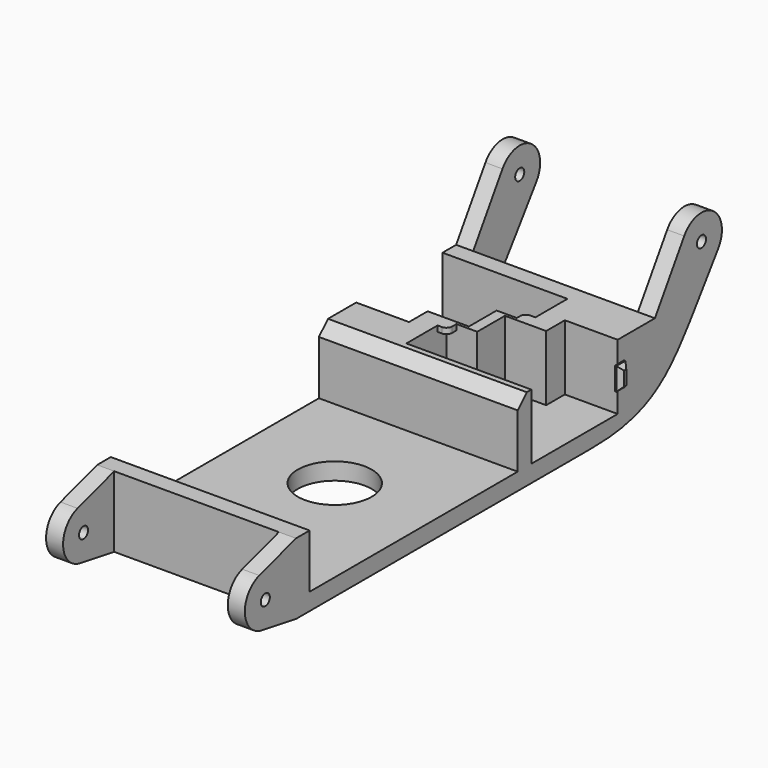
from build123d import *

# Parameters (mm, degrees)
F0_R      = 6.5
F0_W      = 34.999999702
F0_H      = 3
F0_H_2    = 0.3
F1_DEPTH  = 3
F2_DEPTH  = 9.5
F3_DEPTH  = 11.5
F5_DEPTH  = 3
F7_DEPTH  = 3
F8_R      = 1
F9_DEPTH  = 35.000999702
F11_DEPTH = 1
F13_DEPTH = 1
F14_SIZE  = 0.75
F15_W     = 1.8819853365
F15_H     = 1.731043148
F15_W_2   = 1.7636035271
F15_H_2   = 1.938064149
F16_DEPTH = 1
F18_DEPTH = 36.000999702
F19_R     = 1
F20_SIZE2 = 2
F20_SIZE  = 2


# Not quite as in the source:
# - ends of sketch curves that miss each other by under 0.0002 mm in the source are joined
# - a feature names something its author has since deleted; it is built from what else it names


with BuildPart() as f1:
    # F0 (on Top) → F1 (new body)
    with BuildSketch(Plane.XY):
        Polygon((7.8607099131, 16.1003852367), (-9.6392899379, 16.1003852367), (-9.6392899379, -29.3996147633), (25.3607097641, -29.3996147633), (25.3607097641, 16.1003852367), align=None)
        with Locations((7.8607099131, -2.2867515218)):
            Circle(F0_R, mode=Mode.SUBTRACT)
        with Locations((7.8607099131, -31.1996147633)):
            Rectangle(F0_W, F0_H)
        Polygon((-9.6392899379, 19.1003852367), (-9.6392899379, 16.1003852367), (7.8607099131, 16.1003852367), (25.3607097641, 16.1003852367), (25.3607097641, 19.1003852367), (22.192974557, 19.1003852367), (3.3607097641, 19.1003852367), align=None)
        Polygon((-9.6392899379, 46.3003852367), (-9.6392899379, 43.3003852367), (-6.4715547308, 43.3003852367), (12.3607100621, 43.3003852367), (25.3607097641, 43.3003852367), (25.3607097641, 46.3003852367), align=None)
        with Locations((7.8607099131, -29.5496147633)):
            Rectangle(F0_W, F0_H_2)
        Polygon((16.0607097641, 38.1003852367), (25.3607097641, 38.1003852367), (25.3607097641, 43.3003852367), (12.3607100621, 43.3003852367), (12.3607100621, 35.3003852367), (12.3607100621, 34.5003852367), (7.8607097641, 34.5003852367), (7.8607100621, 33.9926332235), (8.7954637781, 33.9926332235), (16.0607097641, 33.9926332235), align=None)
        Polygon((-9.6392899379, 24.3003852367), (-9.6392899379, 19.1003852367), (3.3607097641, 19.1003852367), (3.3607097641, 27.1003852367), (3.3607097641, 27.9003852367), (7.8607100621, 27.9003852367), (7.8607100621, 28.4081372499), (6.9259563461, 28.4081372499), (-0.3392899379, 28.4081372499), (-0.3392899379, 24.3003852367), align=None)
        Polygon((6.9259563461, 34.5003852367), (6.9259563461, 28.4081372499), (7.8607097641, 28.4081372499), (7.8607100621, 33.9926332235), (7.8607100621, 34.5003852367), align=None)
        Polygon((7.8607100621, 28.4081372499), (7.8607100621, 27.9003852367), (8.7954637781, 27.9003852367), (8.7954637781, 33.9926332235), (7.8607097641, 33.9926332235), align=None)
        Polygon((-9.6392899379, 43.3003852367), (-9.6392899379, 24.3003852367), (-0.3392899379, 24.3003852367), (-0.3392899379, 28.4081372499), (6.9259563461, 28.4081372499), (6.9259563461, 34.5003852367), (7.8607100621, 34.5003852367), (12.3607100621, 34.5003852367), (12.3607100621, 35.3003852367), (12.3607100621, 43.3003852367), (-6.4715547308, 43.3003852367), align=None)
        Polygon((3.3607097641, 27.1003852367), (3.3607097641, 19.1003852367), (22.192974557, 19.1003852367), (25.3607097641, 19.1003852367), (25.3607097641, 38.1003852367), (16.0607097641, 38.1003852367), (16.0607097641, 33.9926332235), (8.7954637781, 33.9926332235), (8.7954637781, 27.9003852367), (7.8607100621, 27.9003852367), (3.3607097641, 27.9003852367), align=None)
    extrude(amount=-F1_DEPTH)

    # F0 (on Top) → F2 (join)
    with BuildSketch(Plane.XY):
        with Locations((7.8607099131, -31.1996147633)):
            Rectangle(F0_W, F0_H)
        Polygon((-9.6392899379, 19.1003852367), (-9.6392899379, 16.1003852367), (7.8607099131, 16.1003852367), (25.3607097641, 16.1003852367), (25.3607097641, 19.1003852367), (22.192974557, 19.1003852367), (3.3607097641, 19.1003852367), align=None)
    extrude(amount=F2_DEPTH)

    # F0 (on Top) → F3 (join)
    with BuildSketch(Plane.XY):
        Polygon((-9.6392899379, 46.3003852367), (-9.6392899379, 43.3003852367), (-6.4715547308, 43.3003852367), (12.3607100621, 43.3003852367), (25.3607097641, 43.3003852367), (25.3607097641, 46.3003852367), align=None)
        Polygon((-9.6392899379, 24.3003852367), (-9.6392899379, 19.1003852367), (3.3607097641, 19.1003852367), (3.3607097641, 27.1003852367), (3.3607097641, 27.9003852367), (7.8607100621, 27.9003852367), (7.8607100621, 28.4081372499), (6.9259563461, 28.4081372499), (-0.3392899379, 28.4081372499), (-0.3392899379, 24.3003852367), align=None)
        Polygon((7.8607100621, 28.4081372499), (7.8607100621, 27.9003852367), (8.7954637781, 27.9003852367), (8.7954637781, 33.9926332235), (7.8607097641, 33.9926332235), align=None)
        Polygon((6.9259563461, 34.5003852367), (6.9259563461, 28.4081372499), (7.8607097641, 28.4081372499), (7.8607100621, 33.9926332235), (7.8607100621, 34.5003852367), align=None)
        Polygon((16.0607097641, 38.1003852367), (25.3607097641, 38.1003852367), (25.3607097641, 43.3003852367), (12.3607100621, 43.3003852367), (12.3607100621, 35.3003852367), (12.3607100621, 34.5003852367), (7.8607097641, 34.5003852367), (7.8607100621, 33.9926332235), (8.7954637781, 33.9926332235), (16.0607097641, 33.9926332235), align=None)
        Polygon((-9.6392899379, 19.1003852367), (-9.6392899379, 16.1003852367), (7.8607099131, 16.1003852367), (25.3607097641, 16.1003852367), (25.3607097641, 19.1003852367), (22.192974557, 19.1003852367), (3.3607097641, 19.1003852367), align=None)
    extrude(amount=F3_DEPTH)

    # F4 (on face) → F5 (join)
    with BuildSketch(Plane.YZ.offset(25.3607097641)):
        Polygon((-32.6996147633, -3), (46.3003852367, -3), (46.3003852367, 11.5), (38.1003852367, 11.5), (38.1003852367, 0), (19.1003852367, 0), (19.1003852367, 11.5), (16.1003852367, 11.5), (16.1003852367, 0), (-29.6996147633, 0), (-29.6996147633, 9.5), (-32.6996147633, 9.5), align=None)
        with BuildLine():
            Line((46.3003852367, 11.5), (46.3003852367, -3))
            Line((46.3003852367, -3), (60.2135883006, 16.6053474951))
            ThreePointArc((60.2135883006, 16.6053474951), (54.0324103863, 15.4756413664), (52.7478740756, 21.6265082006))
            Line((52.7478740756, 21.6265082006), (46.3003852367, 11.5))
        make_face()
        with BuildLine():
            ThreePointArc((52.7478740756, 21.6265082006), (54.0324103863, 15.4756413664), (60.2135883006, 16.6053474951))
            ThreePointArc((60.2135883006, 16.6053474951), (60.8312132136, 17.8429507129), (61.0437823534, 19.2096754909))
            ThreePointArc((61.0437823534, 19.2096754909), (57.8024349564, 23.5300682537), (52.7478740756, 21.6265082006))
        make_face()
        with BuildLine():
            Line((-40.2101505455, -1.7121333681), (-32.6996147633, -3))
            Line((-32.6996147633, -3), (-32.6996147633, 9.5))
            Line((-32.6996147633, 9.5), (-40.7689799002, 7.0253734949))
            ThreePointArc((-40.7689799002, 7.0253734949), (-36.7744645914, 6.3416367755), (-34.9496147633, 2.7231327258))
            ThreePointArc((-34.9496147633, 2.7231327258), (-36.5489606146, -0.7172459612), (-40.2101505455, -1.7121333681))
        make_face()
        with BuildLine():
            ThreePointArc((-40.7689799002, 7.0253734949), (-43.9404391312, 2.4359106929), (-40.2101505455, -1.7121333681))
            ThreePointArc((-40.2101505455, -1.7121333681), (-36.5489606146, -0.7172459612), (-34.9496147633, 2.7231327258))
            ThreePointArc((-34.9496147633, 2.7231327258), (-36.7744645914, 6.3416367755), (-40.7689799002, 7.0253734949))
        make_face()
    extrude(amount=-F5_DEPTH)

    # F6 (on face) → F7 (join)
    with BuildSketch(Plane(origin=(-9.6392899379, 0, 0), x_dir=(0, -1, 0), z_dir=(-1, 0, 0))):
        with BuildLine():
            Line((-60.2135883006, 16.6053474951), (-46.3003852367, -3))
            Line((-46.3003852367, -3), (-46.3003852367, 11.5))
            Line((-46.3003852367, 11.5), (-52.7478740756, 21.6265082006))
            ThreePointArc((-52.7478740756, 21.6265082006), (-59.0551543205, 22.9437096154), (-60.2135883006, 16.6053474951))
        make_face()
        Polygon((-46.3003852367, 11.5), (-46.3003852367, -3), (32.6996147633, -3), (32.6996147633, 9.5), (29.6996147633, 9.5), (29.6996147633, 0), (-16.1003852367, 0), (-16.1003852367, 11.5), (-24.3003852367, 11.5), (-24.3003852367, 0), (-43.3003852367, 0), (-43.3003852367, 11.5), align=None)
        with BuildLine():
            Line((32.6996147633, 9.5), (32.6996147633, -3))
            Line((32.6996147633, -3), (40.2101505455, -1.7121333681))
            ThreePointArc((40.2101505455, -1.7121333681), (43.9404391312, 2.4359106929), (40.7689799002, 7.0253734949))
            Line((40.7689799002, 7.0253734949), (32.6996147633, 9.5))
        make_face()
    extrude(amount=-F7_DEPTH)

    # F8 (on face) → F9 (cut, through all)
    with BuildSketch(Plane(origin=(-9.6392899379, 0, 0), x_dir=(0, -1, 0), z_dir=(-1, 0, 0))):
        with Locations((-56.5437823534, 19.2096754909)):
            Circle(F8_R)
        with Locations((39.4496147633, 2.7231327258)):
            Circle(F8_R)
    extrude(amount=-F9_DEPTH, mode=Mode.SUBTRACT)

    # F10 (on face) → F11 (join)
    with BuildSketch(Plane.YZ.offset(25.3607097641)):
        Polygon((39.4906885922, 7.75), (38.1003852367, 7.75), (38.1003852367, 3.75), (39.4906885922, 3.75), (39.4906885922, 5.75), align=None)
        Polygon((38.1003852367, 3.75), (38.1003852367, 7.75), (37.4906885922, 7.75), (37.4906885922, 5.75), (37.4906885922, 3.75), align=None)
    extrude(amount=F11_DEPTH)

    # F12 (on face) → F13 (join)
    with BuildSketch(Plane(origin=(-9.6392899379, 0, 0), x_dir=(0, -1, 0), z_dir=(-1, 0, 0))):
        Polygon((-22.9083076119, 7.75), (-24.3003852367, 7.75), (-24.3003852367, 3.75), (-22.9083076119, 3.75), (-22.9083076119, 5.75), align=None)
        Polygon((-24.9083076119, 7.75), (-24.9083076119, 5.75), (-24.9083076119, 3.75), (-24.3003852367, 3.75), (-24.3003852367, 7.75), align=None)
    extrude(amount=F13_DEPTH)

    # F14
    f14_edges = [f1.edges().sort_by_distance(p)[0] for p in [
        (-10.63929, 24.908308, 5.75),
        (-10.63929, 22.908308, 5.75),
        (-10.63929, 23.908308, 7.75),
        (-10.63929, 23.908308, 3.75),
        (26.36071, 38.490689, 7.75),
        (26.36071, 37.490689, 5.75),
        (26.36071, 38.490689, 3.75),
        (26.36071, 39.490689, 5.75),
    ]]
    chamfer(f14_edges, length=F14_SIZE)

    # F15 (on face) → F16 (join)
    with BuildSketch(Plane.XY.offset(11.5)):
        with Locations((11.4197173938, 35.3659068108)):
            Rectangle(F15_W, F15_H)
        with Locations((4.2425115276, 26.9313531622)):
            Rectangle(F15_W_2, F15_H_2)
    extrude(amount=-F16_DEPTH)

    # F17 (on face) → F18 (cut, through all)
    with BuildSketch(Plane(origin=(-9.6392899379, 0, 0), x_dir=(0, -1, 0), z_dir=(-1, 0, 0))):
        with BuildLine():
            Line((-56.1974216606, 10.9460940352), (-46.3003852367, -3))
            Line((-46.3003852367, -3), (-32.2360508144, -3))
            add(Edge.make_bspline(
                [(-56.1974216606, 10.9460940352), (-49.7821666885, 1.9062415714), (-46.3003852367, -3), (-32.2360508144, -3)],
                knots=[0, 0, 0, 0, 27.7243725207, 27.7243725207, 27.7243725207, 27.7243725207], degree=3))
        make_face()
    extrude(amount=-F18_DEPTH, mode=Mode.SUBTRACT)

    # F19
    f19_edges = [f1.edges().sort_by_distance(p)[0] for p in [
        (5.124313, 25.962321, 11),
        (10.478725, 36.231428, 11),
    ]]
    fillet(f19_edges, radius=F19_R)

    # F20
    f20_edges = [f1.edges().sort_by_distance(p)[0] for p in [
        (7.86071, 16.100385, 11.5),
    ]]
    chamfer(f20_edges, length=F20_SIZE, length2=F20_SIZE2)


solid = f1.part
